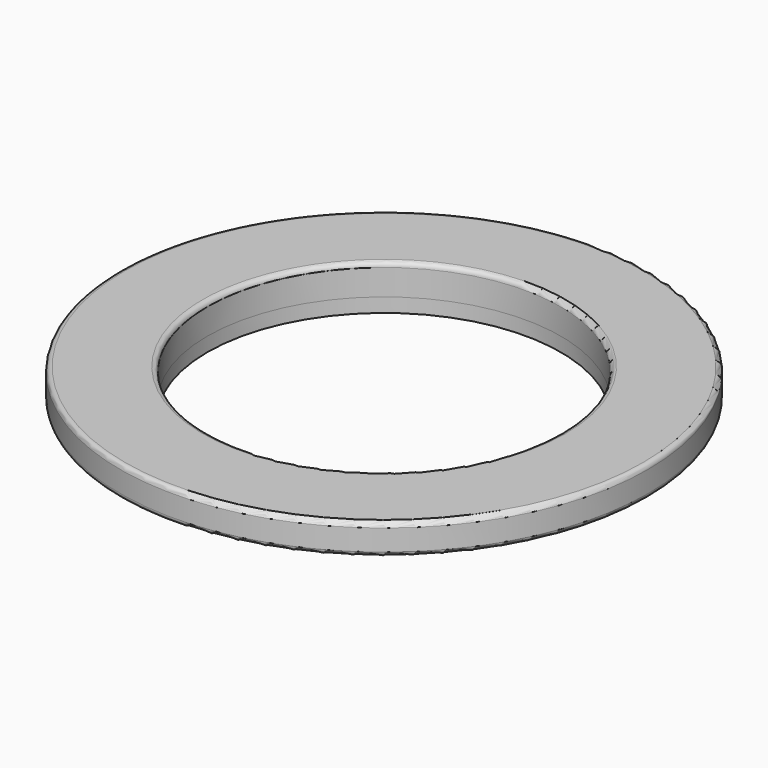
from build123d import *

# Parameters (mm, degrees)
F0_R     = 56
F0_R_2   = 37.5
F1_DEPTH = 6.5
F2_R     = 45
F2_R_2   = 37.5
F3_DEPTH = 3
F4_R     = 1


with BuildPart() as f1:
    # F0 (on Top) → F1 (new body)
    with BuildSketch(Plane.XY):
        Circle(F0_R)
        Circle(F0_R_2, mode=Mode.SUBTRACT)
    extrude(amount=F1_DEPTH)

    # F2 (on Top) → F3 (join)
    with BuildSketch(Plane.XY):
        Circle(F2_R)
        Circle(F2_R_2, mode=Mode.SUBTRACT)
    extrude(amount=-F3_DEPTH)

    # F4
    f4_edges = [f1.edges().sort_by_distance(p)[0] for p in [
        (-56, 0, 6.5),
        (-45, 0, -3),
        (-45, 0, 0),
        (-37.5, 0, 6.5),
        (-56, 0, 0),
    ]]
    fillet(f4_edges, radius=F4_R)


solid = f1.part
